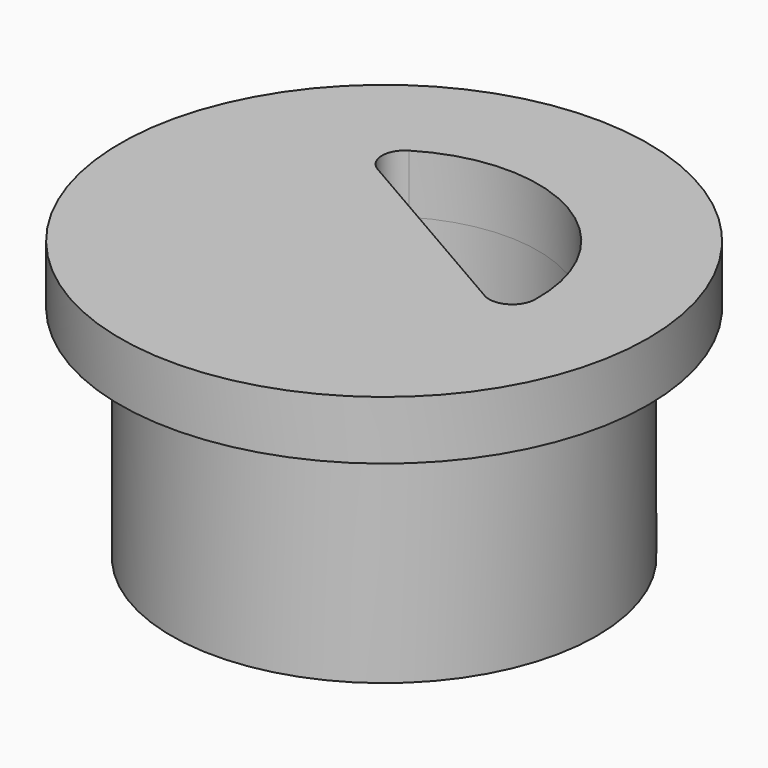
from build123d import *

# Parameters (mm, degrees)
F0_R     = 9.2075
F1_DEPTH = 9.525
F2_R     = 11.43
F3_DEPTH = 2.54
F4_W     = 2.54
F4_H     = 1.016
F5_DEPTH = 2.5
F6_R     = 1


with BuildPart() as f1:
    # F0 (on Top) → F1 (new body)
    with BuildSketch(Plane.XY):
        Circle(F0_R)
        with BuildLine():
            ThreePointArc((-4.7279164178, 4.7013149858), (2.5428501267, 6.1635598061), (6.6675, 0))
            ThreePointArc((6.6675, 0), (6.6092244332, -0.8796070953), (6.4354164178, -1.7438382319))
            ThreePointArc((6.4354164178, -1.7438382319), (6.3636547335, -1.9898378534), (6.2824932589, -2.2328982741))
            ThreePointArc((6.2824932589, -2.2328982741), (-3.33375, -5.7742243797), (-5.0749932589, 4.3243496242))
            ThreePointArc((-5.0749932589, 4.3243496242), (-4.9050774972, 4.5161677335), (-4.7279164178, 4.7013149858))
        make_face(mode=Mode.SUBTRACT)
        with BuildLine():
            Line((6.4354164178, -1.7438382319), (-4.7279164178, 4.7013149858))
            ThreePointArc((-4.7279164178, 4.7013149858), (-4.9050774972, 4.5161677335), (-5.0749932589, 4.3243496242))
            Line((-5.0749932589, 4.3243496242), (6.2824932589, -2.2328982741))
            ThreePointArc((6.2824932589, -2.2328982741), (6.3636547335, -1.9898378534), (6.4354164178, -1.7438382319))
        make_face()
    extrude(amount=F1_DEPTH)

    # F2 (on face) → F3 (join)
    with BuildSketch(Plane.XY.offset(9.525)):
        Circle(F2_R)
        with BuildLine():
            ThreePointArc((-4.7279164178, 4.7013149858), (3.33375, 5.7742243797), (6.4354164178, -1.7438382319))
            Line((6.4354164178, -1.7438382319), (-4.7279164178, 4.7013149858))
        make_face(mode=Mode.SUBTRACT)
    extrude(amount=F3_DEPTH)

    # F4 (on face) → F5 (join)
    with BuildSketch(Plane(origin=(0, 0, 9.525), x_dir=(1, 0, 0), z_dir=(0, 0, -1))):
        with Locations((0, -9.6274932014)):
            Rectangle(F4_W, F4_H)
    extrude(amount=F5_DEPTH)

    # F6
    f6_edges = [f1.edges().sort_by_distance(p)[0] for p in [
        (-4.727916, 4.701315, 6.0325),
        (6.435416, -1.743838, 6.0325),
        (-5.074993, 4.32435, 4.7625),
        (6.282493, -2.232898, 4.7625),
    ]]
    fillet(f6_edges, radius=F6_R)


solid = f1.part
